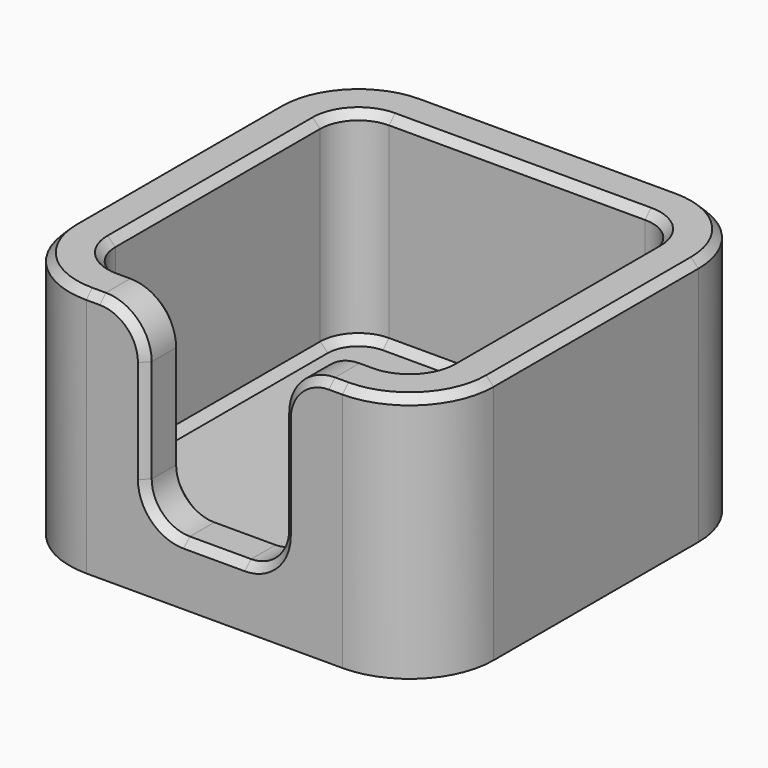
from build123d import *

# Parameters (mm, degrees)
F1_DEPTH = 65
F3_DEPTH = 53
F5_DEPTH = 12
F6_SIZE  = 1.99999


# Not quite as in the source:
# - a fillet or chamfer is up to 0.001 mm smaller than in the source, because OpenCascade refuses the exact size


with BuildPart() as f1:
    # F0 (on Top) → F1 (new body)
    with BuildSketch(Plane.XY):
        with BuildLine():
            Line((55.5, -33.5), (55.5, 33.5))
            ThreePointArc((55.5, 33.5), (49.0563491861, 49.0563491861), (33.5, 55.5))
            Line((33.5, 55.5), (-33.5, 55.5))
            ThreePointArc((-33.5, 55.5), (-49.0563491861, 49.0563491861), (-55.5, 33.5))
            Line((-55.5, 33.5), (-55.5, -33.5))
            ThreePointArc((-55.5, -33.5), (-49.0563491861, -49.0563491861), (-33.5, -55.5))
            Line((-33.5, -55.5), (33.5, -55.5))
            ThreePointArc((33.5, -55.5), (49.0563491861, -49.0563491861), (55.5, -33.5))
        make_face()
    extrude(amount=F1_DEPTH)

    # F2 (on face) → F3 (cut, through all)
    with BuildSketch(Plane.XY.offset(65)):
        with BuildLine():
            Line((33.5, 43.5), (-33.5, 43.5))
            ThreePointArc((-33.5, 43.5), (-40.5710678119, 40.5710678119), (-43.5, 33.5))
            Line((-43.5, 33.5), (-43.5, -33.5))
            ThreePointArc((-43.5, -33.5), (-40.5710678119, -40.5710678119), (-33.5, -43.5))
            Line((-33.5, -43.5), (33.5, -43.5))
            ThreePointArc((33.5, -43.5), (40.5710678119, -40.5710678119), (43.5, -33.5))
            Line((43.5, -33.5), (43.5, 33.5))
            ThreePointArc((43.5, 33.5), (40.5710678119, 40.5710678119), (33.5, 43.5))
        make_face()
    extrude(amount=-F3_DEPTH, mode=Mode.SUBTRACT)

    # F4 (on face) → F5 (cut, through all)
    with BuildSketch(Plane.XZ.offset(55.5)):
        with BuildLine():
            ThreePointArc((-30, 65), (-21.5147186258, 61.4852813742), (-18, 53))
            Line((-18, 53), (-18, 26))
            ThreePointArc((-18, 26), (-15.0710678119, 18.9289321881), (-8, 16))
            Line((-8, 16), (8, 16))
            ThreePointArc((8, 16), (15.0710678119, 18.9289321881), (18, 26))
            Line((18, 26), (18, 53))
            ThreePointArc((18, 53), (21.5147186258, 61.4852813742), (30, 65))
            Line((30, 65), (-30, 65))
        make_face()
    extrude(amount=-F5_DEPTH, mode=Mode.SUBTRACT)

    # F6 (size 2 in the source; OpenCascade refuses exactly that, so slightly less here)
    f6_edges = [f1.edges().sort_by_distance(p)[0] for p in [
        (55.5, 0, 65),
        (-43.5, 0, 65),
        (0, 43.5, 12),
        (-40.571068, 40.571068, 12),
        (-43.5, 0, 12),
        (-40.571068, -40.571068, 12),
        (0, -43.5, 12),
        (40.571068, -40.571068, 12),
        (43.5, 0, 12),
        (40.571068, 40.571068, 12),
    ]]
    chamfer(f6_edges, length=F6_SIZE)


solid = f1.part
